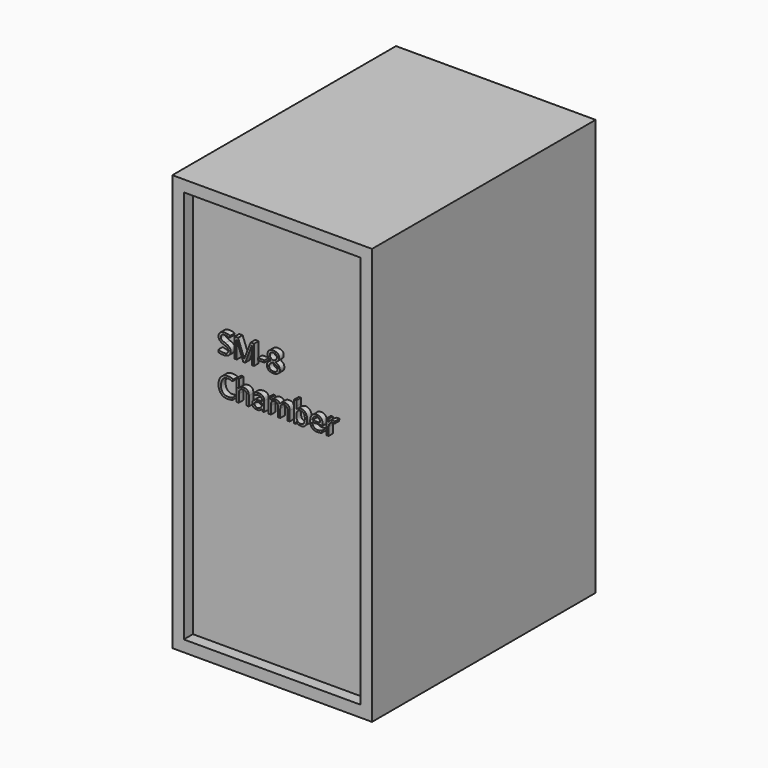
from build123d import *

# Parameters (mm, degrees)
F0_W         = 889
F0_H         = 1244.6
F1_DEPTH     = 1854.2
F2_W         = 787.4
F2_H         = 1752.6
F3_DEPTH     = 50.8
F4_TEXT_SIZE = 122.2343168147
F5_DEPTH     = 25.4


# Not quite as in the source:
# - Text() gives the source's letters only with a copy of the font that has no kerning and outlines rounded to 1/6400 em; it was checked with that copy


with BuildPart() as f1:
    # F0 (on Top) → F1 (new body)
    with BuildSketch(Plane.XY):
        Rectangle(F0_W, F0_H)
    extrude(amount=F1_DEPTH)

    # F2 (on face) → F3 (cut)
    with BuildSketch(Plane.XZ.offset(622.3)):
        with Locations((0, 927.1)):
            Rectangle(F2_W, F2_H)
    extrude(amount=-F3_DEPTH, mode=Mode.SUBTRACT)

    # F4 (on face) → F5 (join)
    with BuildSketch(Plane.XZ.offset(571.5)):
        with Locations((-266.7, 1207.3912918934)):
            Text('SM-8', F4_TEXT_SIZE, font='Open Sans', text_align=(TextAlign.LEFT, TextAlign.BOTTOM))
        with Locations((-266.7, 1041.1526210255)):
            Text('Chamber', F4_TEXT_SIZE, font='Open Sans', text_align=(TextAlign.LEFT, TextAlign.BOTTOM))
    extrude(amount=F5_DEPTH)


solid = f1.part
